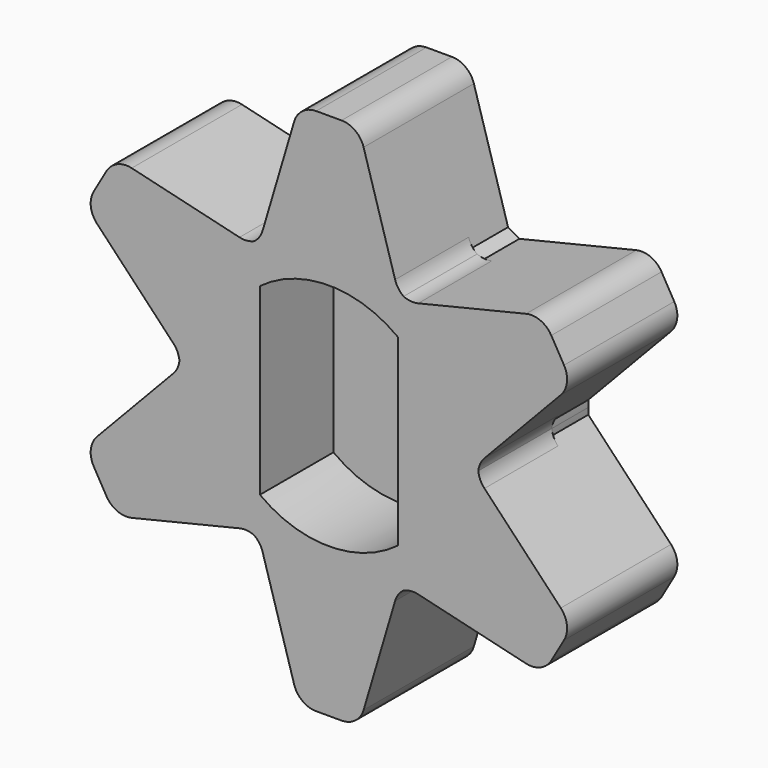
from build123d import *

# Parameters (mm, degrees)
F1_DEPTH    = 2.54
F2_T1_DEPTH = 2.54
F4_DEPTH    = 25.4
F5_DEPTH    = 1.27


# Not quite as in the source:
# - a fillet or chamfer that OpenCascade refuses, or shapes differently, is made with other operations: its cross-section is extruded or revolved along the edge and cut away or added


with BuildPart() as f1:
    # F0 (on Front) → F1 (new body)
    with BuildSketch(Plane.XZ):
        with BuildLine():
            ThreePointArc((4.1235287664, -0.1810159177), (4.1265070722, -0.090529737), (4.1275, 0))
            ThreePointArc((4.1275, 0), (4.1265070722, 0.090529737), (4.1235287664, 0.1810159177))
            ThreePointArc((4.1235287664, 0.1810159177), (3.5745198541, 2.06375), (2.2185287664, 3.4805727061))
            ThreePointArc((2.2185287664, 3.4805727061), (2.06375, 3.5745198541), (1.905, 3.6615886238))
            ThreePointArc((1.905, 3.6615886238), (0, 4.1275), (-1.905, 3.6615886238))
            ThreePointArc((-1.905, 3.6615886238), (-2.06375, 3.5745198541), (-2.2185287664, 3.4805727061))
            ThreePointArc((-2.2185287664, 3.4805727061), (-3.5745198541, 2.06375), (-4.1235287664, 0.1810159177))
            ThreePointArc((-4.1235287664, 0.1810159177), (-4.1275, 0), (-4.1235287664, -0.1810159177))
            ThreePointArc((-4.1235287664, -0.1810159177), (-3.5745198541, -2.06375), (-2.2185287664, -3.4805727061))
            ThreePointArc((-2.2185287664, -3.4805727061), (-2.06375, -3.5745198541), (-1.905, -3.6615886238))
            ThreePointArc((-1.905, -3.6615886238), (0, -4.1275), (1.905, -3.6615886238))
            ThreePointArc((1.905, -3.6615886238), (2.06375, -3.5745198541), (2.2185287664, -3.4805727061))
            ThreePointArc((2.2185287664, -3.4805727061), (3.5745198541, -2.06375), (4.1235287664, -0.1810159177))
        make_face()
        with BuildLine():
            ThreePointArc((2.2185287664, 3.4805727061), (3.5745198541, 2.06375), (4.1235287664, 0.1810159177))
            Line((4.1235287664, 0.1810159177), (6.4106736138, 2.5923984851))
            ThreePointArc((6.4106736138, 2.5923984851), (6.5805571254, 2.9548302166), (6.4998752479, 3.3468858277))
            Line((6.4998752479, 3.3468858277), (6.1484257743, 3.9556141723))
            ThreePointArc((6.1484257743, 3.9556141723), (5.8492365942, 4.2215145333), (5.4504197518, 4.2556069624))
            Line((5.4504197518, 4.2556069624), (2.2185287664, 3.4805727061))
        make_face()
        with BuildLine():
            Line((6.4106736138, -2.5923984851), (4.1235287664, -0.1810159177))
            ThreePointArc((4.1235287664, -0.1810159177), (3.5745198541, -2.06375), (2.2185287664, -3.4805727061))
            Line((2.2185287664, -3.4805727061), (5.4504197518, -4.2556069624))
            ThreePointArc((5.4504197518, -4.2556069624), (5.8492365942, -4.2215145333), (6.1484257743, -3.9556141723))
            Line((6.1484257743, -3.9556141723), (6.4998752479, -3.3468858277))
            ThreePointArc((6.4998752479, -3.3468858277), (6.5805571254, -2.9548302166), (6.4106736138, -2.5923984851))
        make_face()
        with BuildLine():
            ThreePointArc((-1.905, 3.6615886238), (0, 4.1275), (1.905, 3.6615886238))
            Line((1.905, 3.6615886238), (0.9602538621, 6.8480054475))
            ThreePointArc((0.9602538621, 6.8480054475), (0.7313205312, 7.17634475), (0.3514494736, 7.3025))
            Line((0.3514494736, 7.3025), (-0.3514494736, 7.3025))
            ThreePointArc((-0.3514494736, 7.3025), (-0.7313205312, 7.17634475), (-0.9602538621, 6.8480054475))
            Line((-0.9602538621, 6.8480054475), (-1.905, 3.6615886238))
        make_face()
        with BuildLine():
            Line((0.9602538621, -6.8480054475), (1.905, -3.6615886238))
            ThreePointArc((1.905, -3.6615886238), (0, -4.1275), (-1.905, -3.6615886238))
            Line((-1.905, -3.6615886238), (-0.9602538621, -6.8480054475))
            ThreePointArc((-0.9602538621, -6.8480054475), (-0.7313205312, -7.17634475), (-0.3514494736, -7.3025))
            Line((-0.3514494736, -7.3025), (0.3514494736, -7.3025))
            ThreePointArc((0.3514494736, -7.3025), (0.7313205312, -7.17634475), (0.9602538621, -6.8480054475))
        make_face()
        with BuildLine():
            ThreePointArc((-4.1235287664, 0.1810159177), (-3.5745198541, 2.06375), (-2.2185287664, 3.4805727061))
            Line((-2.2185287664, 3.4805727061), (-5.4504197518, 4.2556069624))
            ThreePointArc((-5.4504197518, 4.2556069624), (-5.8492365942, 4.2215145333), (-6.1484257743, 3.9556141723))
            Line((-6.1484257743, 3.9556141723), (-6.4998752479, 3.3468858277))
            ThreePointArc((-6.4998752479, 3.3468858277), (-6.5805571254, 2.9548302166), (-6.4106736138, 2.5923984851))
            Line((-6.4106736138, 2.5923984851), (-4.1235287664, 0.1810159177))
        make_face()
        with BuildLine():
            Line((-5.4504197518, -4.2556069624), (-2.2185287664, -3.4805727061))
            ThreePointArc((-2.2185287664, -3.4805727061), (-3.5745198541, -2.06375), (-4.1235287664, -0.1810159177))
            Line((-4.1235287664, -0.1810159177), (-6.4106736138, -2.5923984851))
            ThreePointArc((-6.4106736138, -2.5923984851), (-6.5805571254, -2.9548302166), (-6.4998752479, -3.3468858277))
            Line((-6.4998752479, -3.3468858277), (-6.1484257743, -3.9556141723))
            ThreePointArc((-6.1484257743, -3.9556141723), (-5.8492365942, -4.2215145333), (-5.4504197518, -4.2556069624))
        make_face()
    extrude(amount=F1_DEPTH)

    # F2: fillet of radius 0.635 on 12 edges, made by hand

    # F2_s2 → F2_t1 (join)
    with BuildSketch(Plane.XZ):
        with BuildLine():
            ThreePointArc((-4.3012819504, 0.3684246555), (-4.1738908411, 0.1709055432), (-4.1270722547, -0.0594209954))
            ThreePointArc((-4.1270722547, -0.0594209954), (-4.1270518266, 0.0608232715), (-4.1235287664, 0.1810159177))
            Line((-4.1235287664, 0.1810159177), (-4.3012819504, 0.3684246555))
        make_face()
        with BuildLine():
            ThreePointArc((-4.1270722547, 0.0594209954), (-4.1738908411, -0.1709055432), (-4.3012819504, -0.3684246555))
            Line((-4.3012819504, -0.3684246555), (-4.1235287664, -0.1810159177))
            ThreePointArc((-4.1235287664, -0.1810159177), (-4.1270518266, -0.0608232715), (-4.1270722547, 0.0594209954))
        make_face()
        with BuildLine():
            ThreePointArc((-1.8315758641, 3.9092317656), (-1.9389368785, 3.7001482727), (-2.1149962189, 3.5444389181))
            ThreePointArc((-2.1149962189, 3.5444389181), (-2.010851415, 3.6045433603), (-1.905, 3.6615886238))
            Line((-1.905, 3.6615886238), (-1.8315758641, 3.9092317656))
        make_face()
        with BuildLine():
            ThreePointArc((4.3012819504, -0.3684246555), (4.1738908411, -0.1709055432), (4.1270722547, 0.0594209954))
            ThreePointArc((4.1270722547, 0.0594209954), (4.1270518266, -0.0608232715), (4.1235287664, -0.1810159177))
            Line((4.1235287664, -0.1810159177), (4.3012819504, -0.3684246555))
        make_face()
        with BuildLine():
            ThreePointArc((2.0120760358, -3.6038599135), (2.2349539626, -3.5292427294), (2.4697060863, -3.5408071101))
            Line((2.4697060863, -3.5408071101), (2.2185287664, -3.4805727061))
            ThreePointArc((2.2185287664, -3.4805727061), (2.1162004116, -3.5437200888), (2.0120760358, -3.6038599135))
        make_face()
        with BuildLine():
            ThreePointArc((1.8315758641, -3.9092317657), (1.9389368785, -3.7001482727), (2.1149962189, -3.5444389181))
            ThreePointArc((2.1149962189, -3.5444389181), (2.010851415, -3.6045433603), (1.905, -3.6615886238))
            Line((1.905, -3.6615886238), (1.8315758641, -3.9092317657))
        make_face()
        with BuildLine():
            ThreePointArc((-2.1149962189, -3.5444389181), (-1.9389368785, -3.7001482727), (-1.8315758641, -3.9092317657))
            Line((-1.8315758641, -3.9092317657), (-1.905, -3.6615886238))
            ThreePointArc((-1.905, -3.6615886238), (-2.010851415, -3.6045433603), (-2.1149962189, -3.5444389181))
        make_face()
        with BuildLine():
            ThreePointArc((-2.4697060863, -3.5408071101), (-2.2349539626, -3.5292427294), (-2.0120760358, -3.6038599135))
            ThreePointArc((-2.0120760358, -3.6038599135), (-2.1162004116, -3.5437200888), (-2.2185287664, -3.4805727061))
            Line((-2.2185287664, -3.4805727061), (-2.4697060863, -3.5408071101))
        make_face()
        with BuildLine():
            ThreePointArc((-2.0120760358, 3.6038599135), (-2.2349539626, 3.5292427294), (-2.4697060863, 3.5408071101))
            Line((-2.4697060863, 3.5408071101), (-2.2185287664, 3.4805727061))
            ThreePointArc((-2.2185287664, 3.4805727061), (-2.1162004116, 3.5437200888), (-2.0120760358, 3.6038599135))
        make_face()
        with BuildLine():
            ThreePointArc((2.1149962189, 3.5444389181), (1.9389368785, 3.7001482727), (1.8315758641, 3.9092317656))
            Line((1.8315758641, 3.9092317656), (1.905, 3.6615886238))
            ThreePointArc((1.905, 3.6615886238), (2.010851415, 3.6045433603), (2.1149962189, 3.5444389181))
        make_face()
        with BuildLine():
            ThreePointArc((2.0120760358, 3.6038599135), (2.2349539626, 3.5292427294), (2.4697060863, 3.5408071101))
            Line((2.4697060863, 3.5408071101), (2.2185287664, 3.4805727061))
            ThreePointArc((2.2185287664, 3.4805727061), (2.1162004116, 3.5437200888), (2.0120760358, 3.6038599135))
        make_face()
        with BuildLine():
            ThreePointArc((4.1270722547, -0.0594209954), (4.1738908411, 0.1709055432), (4.3012819504, 0.3684246555))
            Line((4.3012819504, 0.3684246555), (4.1235287664, 0.1810159177))
            ThreePointArc((4.1235287664, 0.1810159177), (4.1270518266, 0.0608232715), (4.1270722547, -0.0594209954))
        make_face()
    extrude(amount=F2_T1_DEPTH)

    # F3 (on face) → F4 (cut)
    with BuildSketch(Plane(origin=(0, 0, 0), x_dir=(-1, 0, 0), z_dir=(0, 1, 0))):
        with BuildLine():
            Line((-1.905, 2.54), (-1.905, -2.54))
            ThreePointArc((-1.905, -2.54), (0, -3.175), (1.905, -2.54))
            Line((1.905, -2.54), (1.905, 2.54))
            ThreePointArc((1.905, 2.54), (0, 3.175), (-1.905, 2.54))
        make_face()
    extrude(amount=-F4_DEPTH, mode=Mode.SUBTRACT)

    # F0 (on Front) → F5 (join)
    with BuildSketch(Plane.XZ):
        with BuildLine():
            ThreePointArc((4.1235287664, -0.1810159177), (4.1265070722, -0.090529737), (4.1275, 0))
            ThreePointArc((4.1275, 0), (4.1265070722, 0.090529737), (4.1235287664, 0.1810159177))
            ThreePointArc((4.1235287664, 0.1810159177), (3.5745198541, 2.06375), (2.2185287664, 3.4805727061))
            ThreePointArc((2.2185287664, 3.4805727061), (2.06375, 3.5745198541), (1.905, 3.6615886238))
            ThreePointArc((1.905, 3.6615886238), (0, 4.1275), (-1.905, 3.6615886238))
            ThreePointArc((-1.905, 3.6615886238), (-2.06375, 3.5745198541), (-2.2185287664, 3.4805727061))
            ThreePointArc((-2.2185287664, 3.4805727061), (-3.5745198541, 2.06375), (-4.1235287664, 0.1810159177))
            ThreePointArc((-4.1235287664, 0.1810159177), (-4.1275, 0), (-4.1235287664, -0.1810159177))
            ThreePointArc((-4.1235287664, -0.1810159177), (-3.5745198541, -2.06375), (-2.2185287664, -3.4805727061))
            ThreePointArc((-2.2185287664, -3.4805727061), (-2.06375, -3.5745198541), (-1.905, -3.6615886238))
            ThreePointArc((-1.905, -3.6615886238), (0, -4.1275), (1.905, -3.6615886238))
            ThreePointArc((1.905, -3.6615886238), (2.06375, -3.5745198541), (2.2185287664, -3.4805727061))
            ThreePointArc((2.2185287664, -3.4805727061), (3.5745198541, -2.06375), (4.1235287664, -0.1810159177))
        make_face()
        with BuildLine():
            ThreePointArc((2.2185287664, 3.4805727061), (3.5745198541, 2.06375), (4.1235287664, 0.1810159177))
            Line((4.1235287664, 0.1810159177), (6.4106736138, 2.5923984851))
            ThreePointArc((6.4106736138, 2.5923984851), (6.5805571254, 2.9548302166), (6.4998752479, 3.3468858277))
            Line((6.4998752479, 3.3468858277), (6.1484257743, 3.9556141723))
            ThreePointArc((6.1484257743, 3.9556141723), (5.8492365942, 4.2215145333), (5.4504197518, 4.2556069624))
            Line((5.4504197518, 4.2556069624), (2.2185287664, 3.4805727061))
        make_face()
        with BuildLine():
            Line((6.4106736138, -2.5923984851), (4.1235287664, -0.1810159177))
            ThreePointArc((4.1235287664, -0.1810159177), (3.5745198541, -2.06375), (2.2185287664, -3.4805727061))
            Line((2.2185287664, -3.4805727061), (5.4504197518, -4.2556069624))
            ThreePointArc((5.4504197518, -4.2556069624), (5.8492365942, -4.2215145333), (6.1484257743, -3.9556141723))
            Line((6.1484257743, -3.9556141723), (6.4998752479, -3.3468858277))
            ThreePointArc((6.4998752479, -3.3468858277), (6.5805571254, -2.9548302166), (6.4106736138, -2.5923984851))
        make_face()
        with BuildLine():
            ThreePointArc((-1.905, 3.6615886238), (0, 4.1275), (1.905, 3.6615886238))
            Line((1.905, 3.6615886238), (0.9602538621, 6.8480054475))
            ThreePointArc((0.9602538621, 6.8480054475), (0.7313205312, 7.17634475), (0.3514494736, 7.3025))
            Line((0.3514494736, 7.3025), (-0.3514494736, 7.3025))
            ThreePointArc((-0.3514494736, 7.3025), (-0.7313205312, 7.17634475), (-0.9602538621, 6.8480054475))
            Line((-0.9602538621, 6.8480054475), (-1.905, 3.6615886238))
        make_face()
        with BuildLine():
            Line((0.9602538621, -6.8480054475), (1.905, -3.6615886238))
            ThreePointArc((1.905, -3.6615886238), (0, -4.1275), (-1.905, -3.6615886238))
            Line((-1.905, -3.6615886238), (-0.9602538621, -6.8480054475))
            ThreePointArc((-0.9602538621, -6.8480054475), (-0.7313205312, -7.17634475), (-0.3514494736, -7.3025))
            Line((-0.3514494736, -7.3025), (0.3514494736, -7.3025))
            ThreePointArc((0.3514494736, -7.3025), (0.7313205312, -7.17634475), (0.9602538621, -6.8480054475))
        make_face()
        with BuildLine():
            ThreePointArc((-4.1235287664, 0.1810159177), (-3.5745198541, 2.06375), (-2.2185287664, 3.4805727061))
            Line((-2.2185287664, 3.4805727061), (-5.4504197518, 4.2556069624))
            ThreePointArc((-5.4504197518, 4.2556069624), (-5.8492365942, 4.2215145333), (-6.1484257743, 3.9556141723))
            Line((-6.1484257743, 3.9556141723), (-6.4998752479, 3.3468858277))
            ThreePointArc((-6.4998752479, 3.3468858277), (-6.5805571254, 2.9548302166), (-6.4106736138, 2.5923984851))
            Line((-6.4106736138, 2.5923984851), (-4.1235287664, 0.1810159177))
        make_face()
        with BuildLine():
            Line((-5.4504197518, -4.2556069624), (-2.2185287664, -3.4805727061))
            ThreePointArc((-2.2185287664, -3.4805727061), (-3.5745198541, -2.06375), (-4.1235287664, -0.1810159177))
            Line((-4.1235287664, -0.1810159177), (-6.4106736138, -2.5923984851))
            ThreePointArc((-6.4106736138, -2.5923984851), (-6.5805571254, -2.9548302166), (-6.4998752479, -3.3468858277))
            Line((-6.4998752479, -3.3468858277), (-6.1484257743, -3.9556141723))
            ThreePointArc((-6.1484257743, -3.9556141723), (-5.8492365942, -4.2215145333), (-5.4504197518, -4.2556069624))
        make_face()
    extrude(amount=-F5_DEPTH)


solid = f1.part
